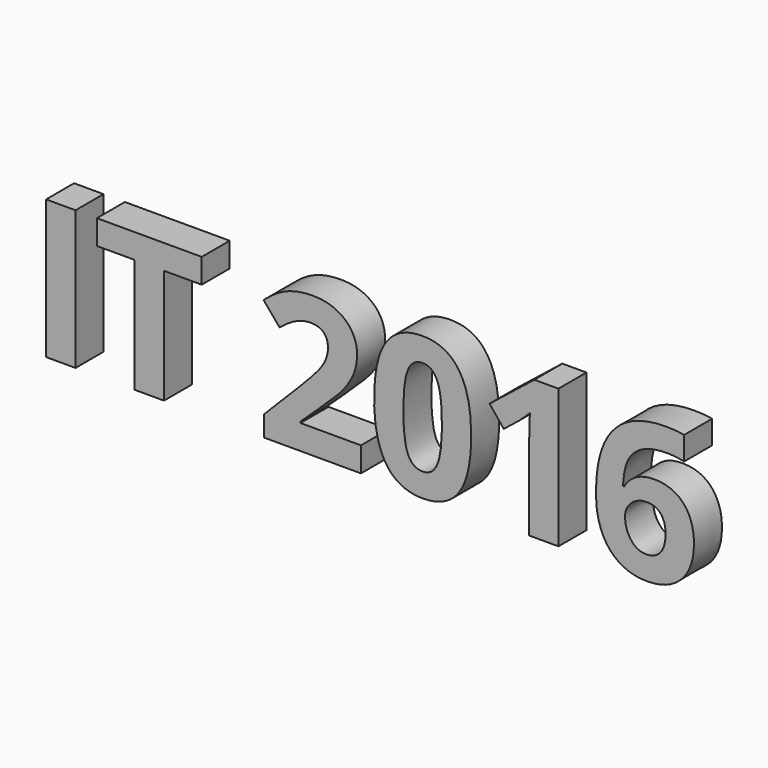
from build123d import *

# Parameters (mm, degrees)
F0_TEXT_SIZE = 2.7777777778
F1_DEPTH     = 0.5


# Not quite as in the source:
# - Text() gives the source's letters only with a copy of the font that has no kerning and outlines rounded to 1/6400 em; it was checked with that copy


with BuildPart() as f1:
    # F0 (on Front) → F1 (new body)
    with BuildSketch(Plane.XZ):
        with Locations((0, 0)):
            Text('IT 2016', F0_TEXT_SIZE, font='Open Sans', font_style=FontStyle.BOLD, text_align=(TextAlign.LEFT, TextAlign.BOTTOM))
    extrude(amount=F1_DEPTH)


solid = f1.part
